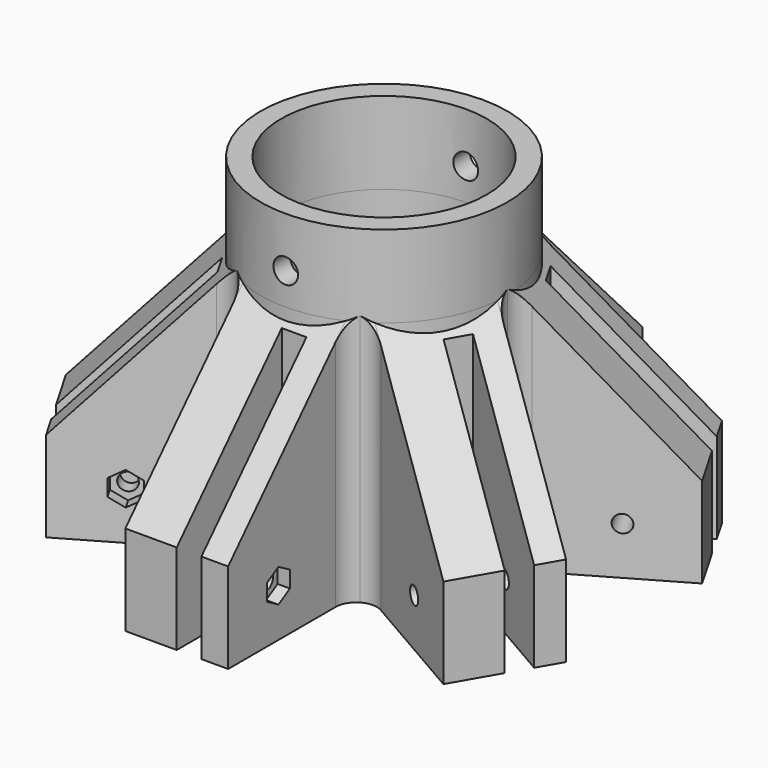
from build123d import *

# Parameters (mm, degrees)
F0_R          = 30
F1_DEPTH      = 60
F2_W          = 25
F2_H          = 60
F3_DEPTH      = 63
F5_DEPTH      = 25
F6_W          = 6
F6_H          = 32.6840691268
F5_FACE_W     = 25
F5_FACE_H     = 52.1894276986
F7_DEPTH      = 114.6
F8_R          = 2.1
F9_DEPTH      = 3
F10_D         = 4.2
F11_COUNT     = 6
F12_R         = 25.0000537328
F13_DEPTH     = 60.001
F14_DEPTH     = 20
F15_T4_DEPTH  = 67.5977721147
F15_T9_DEPTH  = 67.5977721147
F15_T14_DEPTH = 67.5977721147
F15_T19_DEPTH = 67.5977721147
F15_T24_DEPTH = 67.5977721147
F15_T29_DEPTH = 67.5977721147
F15_T34_DEPTH = 67.5977721147
F15_T39_DEPTH = 67.5977721147
F15_T44_DEPTH = 67.5977721147
F15_T49_DEPTH = 67.5977721147
F15_T54_DEPTH = 67.5977721147
F15_T59_DEPTH = 67.5977721147
F16_R         = 3
F17_DEPTH     = 38.3


# Not quite as in the source:
# - a fillet or chamfer that OpenCascade refuses, or shapes differently, is made with other operations: its cross-section is extruded or revolved along the edge and cut away or added
# - after a boolean that leaves OpenCascade's solid faulty, fix() repairs it
# - a feature names something its author has since deleted; it is built from what else it names


with BuildPart() as f1:
    # F0 (on Top) → F1 (new body)
    with BuildSketch(Plane.XY):
        Circle(F0_R)
    extrude(amount=F1_DEPTH)

    # F2 (on Front) → F3 (join)
    with BuildSketch(Plane.XZ):
        with Locations((0, 30)):
            Rectangle(F2_W, F2_H)
    extrude(amount=F3_DEPTH)

    # F4 (on face) → F5 (cut)
    with BuildSketch(Plane.YZ.offset(12.5)):
        Polygon((-63, 21.9575148076), (-27.2717802866, 60), (-63, 60), align=None)
    extrude(amount=-F5_DEPTH, mode=Mode.SUBTRACT)

    # F6 (on Top) + F5_face (on face) → F7 (cut)
    with BuildSketch(Plane.XY):
        with Locations((3, -47.4198181182)):
            Rectangle(F6_W, F6_H)
    with BuildSketch(Plane(origin=(0, -45.1358901433, 40.9787574038), x_dir=(1, 0, 0), z_dir=(0, -0.7289308749, 0.6845873061))):
        Rectangle(F5_FACE_W, F5_FACE_H)
    extrude(amount=F7_DEPTH, dir=(0, 0, 1), mode=Mode.SUBTRACT)

    # F8 (on face) → F9 (cut)
    with BuildSketch(Plane.YZ.offset(12.5)):
        Polygon((-44.2129718781, 9.5931431661), (-44.2129718781, 13.6345950504), (-47.7129718781, 15.6553209926), (-51.2129718781, 13.6345950504), (-51.2129718781, 9.5931431661), (-47.7129718781, 7.5724172239), align=None)
        with Locations((-47.7129718781, 11.6138691083)):
            Circle(F8_R, mode=Mode.SUBTRACT)
    extrude(amount=-F9_DEPTH, mode=Mode.SUBTRACT)

    # F10 (through all)
    with Locations(Plane.YZ.offset(12.5)):
        with Locations((-47.7129718781, 11.6138691083)):
            Hole(F10_D / 2)

    # F11: F1 ×6 about axis
    f11_axis = Axis((0, 0, 0), (0, 0, -1))


with BuildPart() as f1_1:
    add(f1.part)
    for i in range(1, F11_COUNT):
        add(f1.part.rotate(f11_axis, i * 360 / F11_COUNT))

    # F12 (on face) → F13 (cut, through all)
    with BuildSketch(Plane.XY.offset(60)):
        Circle(F12_R)
    extrude(amount=-F13_DEPTH, mode=Mode.SUBTRACT)

    # F14 (add): a face of the model
    f14_faces = [f1_1.faces().sort_by_distance(p)[0] for p in [
        (-14.5757359313, -25.2459151907, 60),
    ]]
    extrude(f14_faces, amount=F14_DEPTH)

    # F15: fillet of radius 5 on 12 edges, made by hand


with BuildPart() as f15_tool2:
    # F15_s3 → F15_t4 (new body)
    with BuildSketch(Plane.XY.offset(67.5977721147)):
        with BuildLine():
            ThreePointArc((15, -25.9807621135), (13.1698729811, -27.8108891325), (12.5, -30.3108891325))
            Line((12.5, -30.3108891325), (12.5, -27.2717802866))
            ThreePointArc((12.5, -27.2717802866), (13.7651437327, -26.6555963734), (15, -25.9807621135))
        make_face()
    extrude(amount=-F15_T4_DEPTH)

    split(bisect_by=Plane(origin=(0, -44.4316031845, 41.7286639599), x_dir=(1, 0, 0), z_dir=(0, 0.7289308749, -0.6845873061)), keep=Keep.TOP)


with BuildPart() as f1_2:
    add(f1_1.part)

    # F15_t1: union F15_tool2
    add(f15_tool2.part)


with BuildPart() as f15_tool7:
    # F15_s8 → F15_t9 (new body)
    with BuildSketch(Plane.XY.offset(67.5977721147)):
        with BuildLine():
            ThreePointArc((-12.5, -30.3108891325), (-13.1698729811, -27.8108891325), (-15, -25.9807621135))
            ThreePointArc((-15, -25.9807621135), (-13.7651437327, -26.6555963734), (-12.5, -27.2717802866))
            Line((-12.5, -27.2717802866), (-12.5, -30.3108891325))
        make_face()
    extrude(amount=-F15_T9_DEPTH)

    split(bisect_by=Plane(origin=(0, -44.4316031845, 41.7286639599), x_dir=(1, 0, 0), z_dir=(0, 0.7289308749, -0.6845873061)), keep=Keep.TOP)


with BuildPart() as f1_3:
    add(f1_2.part)

    # F15_t6: union F15_tool7
    add(f15_tool7.part)


with BuildPart() as f15_tool12:
    # F15_s13 → F15_t14 (new body)
    with BuildSketch(Plane.XY.offset(67.5977721147)):
        with BuildLine():
            ThreePointArc((-15, -25.9807621135), (-17.5, -25.3108891325), (-20, -25.9807621135))
            Line((-20, -25.9807621135), (-17.3680545346, -24.4612076906))
            ThreePointArc((-17.3680545346, -24.4612076906), (-16.201851746, -25.2487623459), (-15, -25.9807621135))
        make_face()
    extrude(amount=-F15_T14_DEPTH)

    split(bisect_by=Plane(origin=(-38.4788970886, -22.2158015922, 41.7286639599), x_dir=(-0.5, 0.8660254038, 0), z_dir=(0.6312726553, 0.3644654374, -0.6845873061)), keep=Keep.TOP)


with BuildPart() as f1_4:
    add(f1_3.part)

    # F15_t11: union F15_tool12
    add(f15_tool12.part)


with BuildPart() as f15_tool17:
    # F15_s18 → F15_t19 (new body)
    with BuildSketch(Plane.XY.offset(67.5977721147)):
        with BuildLine():
            ThreePointArc((-32.5, -4.3301270189), (-30.6698729811, -2.5), (-30, 0))
            ThreePointArc((-30, 0), (-29.9669954787, -1.4068340274), (-29.8680545346, -2.810572596))
            Line((-29.8680545346, -2.810572596), (-32.5, -4.3301270189))
        make_face()
    extrude(amount=-F15_T19_DEPTH)

    split(bisect_by=Plane(origin=(-38.4788970886, -22.2158015922, 41.7286639599), x_dir=(-0.5, 0.8660254038, 0), z_dir=(0.6312726553, 0.3644654374, -0.6845873061)), keep=Keep.TOP)


with BuildPart() as f1_5:
    add(f1_4.part)

    # F15_t16: union F15_tool17
    add(f15_tool17.part)


with BuildPart() as f15_tool22:
    # F15_s23 → F15_t24 (new body)
    with BuildSketch(Plane.XY.offset(67.5977721147)):
        with BuildLine():
            ThreePointArc((15, -25.9807621135), (17.5, -25.3108891325), (20, -25.9807621135))
            Line((20, -25.9807621135), (17.3680545346, -24.4612076906))
            ThreePointArc((17.3680545346, -24.4612076906), (16.201851746, -25.2487623459), (15, -25.9807621135))
        make_face()
    extrude(amount=-F15_T24_DEPTH)

    split(bisect_by=Plane(origin=(38.4788970886, -22.2158015922, 41.7286639599), x_dir=(-0.5, -0.8660254038, 0), z_dir=(-0.6312726553, 0.3644654374, -0.6845873061)), keep=Keep.TOP)


with BuildPart() as f1_6:
    add(f1_5.part)

    # F15_t21: union F15_tool22
    add(f15_tool22.part)


with BuildPart() as f15_tool27:
    # F15_s28 → F15_t29 (new body)
    with BuildSketch(Plane.XY.offset(67.5977721147)):
        with BuildLine():
            ThreePointArc((30, 0), (30.6698729811, 2.5), (32.5, 4.3301270189))
            Line((32.5, 4.3301270189), (29.8680545346, 2.810572596))
            ThreePointArc((29.8680545346, 2.810572596), (29.9669954787, 1.4068340274), (30, 0))
        make_face()
    extrude(amount=-F15_T29_DEPTH)

    split(bisect_by=Plane(origin=(38.4788970886, 22.2158015922, 41.7286639599), x_dir=(0.5, -0.8660254038, 0), z_dir=(-0.6312726553, -0.3644654374, -0.6845873061)), keep=Keep.TOP)


with BuildPart() as f1_7:
    add(f1_6.part)

    # F15_t26: union F15_tool27
    add(f15_tool27.part)


with BuildPart() as f15_tool32:
    # F15_s33 → F15_t34 (new body)
    with BuildSketch(Plane.XY.offset(67.5977721147)):
        with BuildLine():
            ThreePointArc((30, 0), (30.6698729811, -2.5), (32.5, -4.3301270189))
            Line((32.5, -4.3301270189), (29.8680545346, -2.810572596))
            ThreePointArc((29.8680545346, -2.810572596), (29.9669954787, -1.4068340274), (30, 0))
        make_face()
    extrude(amount=-F15_T34_DEPTH)

    split(bisect_by=Plane(origin=(38.4788970886, -22.2158015922, 41.7286639599), x_dir=(-0.5, -0.8660254038, 0), z_dir=(-0.6312726553, 0.3644654374, -0.6845873061)), keep=Keep.TOP)


with BuildPart() as f1_8:
    add(f1_7.part)

    # F15_t31: union F15_tool32
    add(f15_tool32.part)


with BuildPart() as f15_tool37:
    # F15_s38 → F15_t39 (new body)
    with BuildSketch(Plane.XY.offset(67.5977721147)):
        with BuildLine():
            ThreePointArc((20, 25.9807621135), (17.5, 25.3108891325), (15, 25.9807621135))
            ThreePointArc((15, 25.9807621135), (16.201851746, 25.2487623459), (17.3680545346, 24.4612076906))
            Line((17.3680545346, 24.4612076906), (20, 25.9807621135))
        make_face()
    extrude(amount=-F15_T39_DEPTH)

    split(bisect_by=Plane(origin=(38.4788970886, 22.2158015922, 41.7286639599), x_dir=(0.5, -0.8660254038, 0), z_dir=(-0.6312726553, -0.3644654374, -0.6845873061)), keep=Keep.TOP)


with BuildPart() as f1_9:
    add(f1_8.part)

    # F15_t36: union F15_tool37
    add(f15_tool37.part)


with BuildPart() as f15_tool42:
    # F15_s43 → F15_t44 (new body)
    with BuildSketch(Plane.XY.offset(67.5977721147)):
        with BuildLine():
            ThreePointArc((15, 25.9807621135), (13.1698729811, 27.8108891325), (12.5, 30.3108891325))
            Line((12.5, 30.3108891325), (12.5, 27.2717802866))
            ThreePointArc((12.5, 27.2717802866), (13.7651437327, 26.6555963734), (15, 25.9807621135))
        make_face()
    extrude(amount=-F15_T44_DEPTH)

    split(bisect_by=Plane(origin=(0, 44.4316031845, 41.7286639599), x_dir=(1, 0, 0), z_dir=(0, -0.7289308749, -0.6845873061)), keep=Keep.TOP)


with BuildPart() as f1_10:
    add(f1_9.part)

    # F15_t41: union F15_tool42
    add(f15_tool42.part)


with BuildPart() as f15_tool47:
    # F15_s48 → F15_t49 (new body)
    with BuildSketch(Plane.XY.offset(67.5977721147)):
        with BuildLine():
            ThreePointArc((-12.5, 30.3108891325), (-13.1698729811, 27.8108891325), (-15, 25.9807621135))
            ThreePointArc((-15, 25.9807621135), (-13.7651437327, 26.6555963734), (-12.5, 27.2717802866))
            Line((-12.5, 27.2717802866), (-12.5, 30.3108891325))
        make_face()
    extrude(amount=-F15_T49_DEPTH)

    split(bisect_by=Plane(origin=(0, 44.4316031845, 41.7286639599), x_dir=(1, 0, 0), z_dir=(0, -0.7289308749, -0.6845873061)), keep=Keep.TOP)


with BuildPart() as f1_11:
    add(f1_10.part)

    # F15_t46: union F15_tool47
    add(f15_tool47.part)


with BuildPart() as f15_tool52:
    # F15_s53 → F15_t54 (new body)
    with BuildSketch(Plane.XY.offset(67.5977721147)):
        with BuildLine():
            ThreePointArc((-15, 25.9807621135), (-17.5, 25.3108891325), (-20, 25.9807621135))
            Line((-20, 25.9807621135), (-17.3680545346, 24.4612076906))
            ThreePointArc((-17.3680545346, 24.4612076906), (-16.201851746, 25.2487623459), (-15, 25.9807621135))
        make_face()
    extrude(amount=-F15_T54_DEPTH)

    split(bisect_by=Plane(origin=(-38.4788970886, 22.2158015922, 41.7286639599), x_dir=(0.5, 0.8660254038, 0), z_dir=(0.6312726553, -0.3644654374, -0.6845873061)), keep=Keep.TOP)


with BuildPart() as f1_12:
    add(f1_11.part)

    # F15_t51: union F15_tool52
    add(f15_tool52.part)


with BuildPart() as f15_tool57:
    # F15_s58 → F15_t59 (new body)
    with BuildSketch(Plane.XY.offset(67.5977721147)):
        with BuildLine():
            ThreePointArc((-32.5, 4.3301270189), (-30.6698729811, 2.5), (-30, 0))
            ThreePointArc((-30, 0), (-29.9669954787, 1.4068340274), (-29.8680545346, 2.810572596))
            Line((-29.8680545346, 2.810572596), (-32.5, 4.3301270189))
        make_face()
    extrude(amount=-F15_T59_DEPTH)

    split(bisect_by=Plane(origin=(-38.4788970886, 22.2158015922, 41.7286639599), x_dir=(0.5, 0.8660254038, 0), z_dir=(0.6312726553, -0.3644654374, -0.6845873061)), keep=Keep.TOP)


with BuildPart() as f1_13:
    add(f1_12.part)

    # F15_t56: union F15_tool57
    add(f15_tool57.part)

    # F16 (on Front) → F17 (cut, symmetric)
    with BuildSketch(Plane.XZ):
        with Locations((0, 67.792750895)):
            Circle(F16_R)
    extrude(amount=F17_DEPTH, both=True, mode=Mode.SUBTRACT)

    add(f1_13.part.fix(), mode=Mode.REPLACE)


solid = f1_13.part
